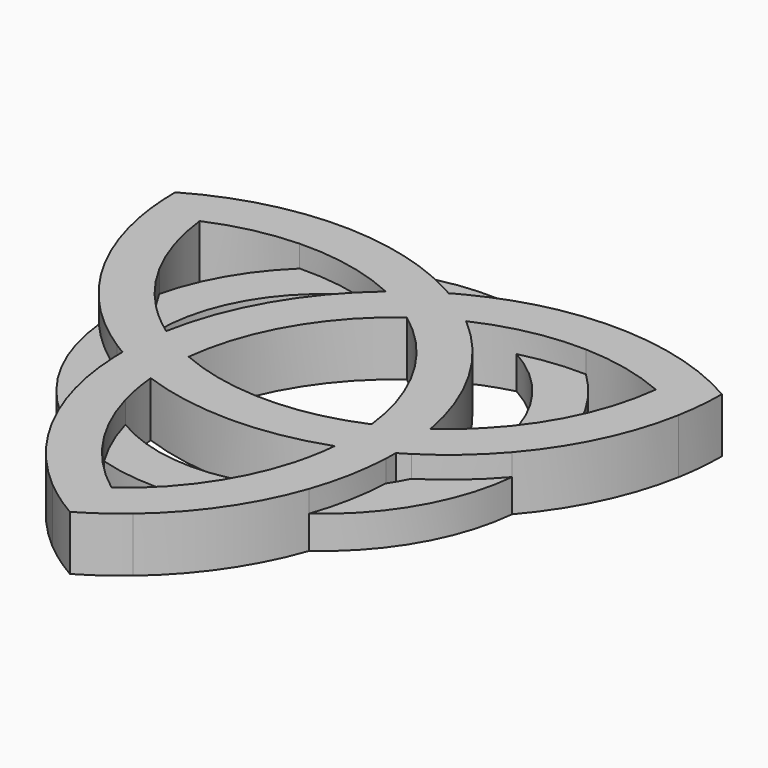
from build123d import *

# Parameters (mm, degrees)
F1_DEPTH = 5
F2_DEPTH = 3


with BuildPart() as f1:
    # F0 (on Top) → F1 (new body)
    with BuildSketch(Plane.XY):
        with BuildLine():
            ThreePointArc((24.5947175074, 9.9504687923), (24.8984732231, 12.1829721649), (25, 14.4337567297))
            ThreePointArc((25, 14.4337567297), (23, 15.4712242442), (20.9147175074, 16.3244157642))
            ThreePointArc((20.9147175074, 16.3244157642), (20.9786685428, 15.3800474736), (21, 14.4337567297))
            ThreePointArc((21, 14.4337567297), (20.9659167777, 13.237791149), (20.8637777457, 12.0457076978))
            ThreePointArc((20.8637777457, 12.0457076978), (22.7827532073, 11.0933643008), (24.5947175074, 9.9504687923))
        make_face()
        with BuildLine():
            ThreePointArc((18.901890558, -1.9283498991), (22.544740222, 3.6293739003), (24.5947175074, 9.9504687923))
            ThreePointArc((24.5947175074, 9.9504687923), (22.7827532073, 11.0933643008), (20.8637777457, 12.0457076978))
            ThreePointArc((20.8637777457, 12.0457076978), (20.0319225906, 8.1312114245), (18.4725923104, 4.4455970728))
            ThreePointArc((18.4725923104, 4.4455970728), (18.8676873768, 2.2383862605), (19, 0))
            ThreePointArc((19, 0), (18.9754567877, -0.9654220315), (18.901890558, -1.9283498991))
        make_face()
        with BuildLine():
            ThreePointArc((13.4505266316, -6.6395280957), (16.3468200119, -4.4813556278), (18.901890558, -1.9283498991))
            ThreePointArc((18.901890558, -1.9283498991), (18.9754567877, -0.9654220315), (19, 0))
            ThreePointArc((19, 0), (18.8676873768, 2.2383862605), (18.4725923104, 4.4455970728))
            ThreePointArc((18.4725923104, 4.4455970728), (16.900090485, 1.9683268696), (14.9976487046, -0.2655811238))
            ThreePointArc((14.9976487046, -0.2655811238), (14.5767441491, -3.5381534747), (13.4505266316, -6.6395280957))
        make_face()
        with BuildLine():
            ThreePointArc((12.5, -7.2168783649), (12.9784741571, -6.9334894324), (13.4505266316, -6.6395280957))
            ThreePointArc((13.4505266316, -6.6395280957), (14.5767441491, -3.5381534747), (14.9976487046, -0.2655811238))
            ThreePointArc((14.9976487046, -0.2655811238), (13.6022734946, -1.5655606237), (12.0947175074, -2.7335904275))
            ThreePointArc((12.0947175074, -2.7335904275), (12.3984732231, -4.9660938001), (12.5, -7.2168783649))
        make_face()
        with BuildLine():
            ThreePointArc((8.4147175074, -9.1075373993), (10.5, -8.2543458793), (12.5, -7.2168783649))
            ThreePointArc((12.5, -7.2168783649), (12.3984732231, -4.9660938001), (12.0947175074, -2.7335904275))
            ThreePointArc((12.0947175074, -2.7335904275), (10.2827532073, -3.876485936), (8.3637777457, -4.8288293329))
            ThreePointArc((8.3637777457, -4.8288293329), (8.4659167777, -6.0209127841), (8.5, -7.2168783649))
            ThreePointArc((8.5, -7.2168783649), (8.4786685428, -8.1631691088), (8.4147175074, -9.1075373993))
        make_face()
        with BuildLine():
            ThreePointArc((-8.4147175074, -9.1075373993), (0, -10.5662432703), (8.4147175074, -9.1075373993))
            ThreePointArc((8.4147175074, -9.1075373993), (8.4786685428, -8.1631691088), (8.5, -7.2168783649))
            ThreePointArc((8.5, -7.2168783649), (8.4659167777, -6.0209127841), (8.3637777457, -4.8288293329))
            ThreePointArc((8.3637777457, -4.8288293329), (0, -6.5662432703), (-8.3637777457, -4.8288293329))
            ThreePointArc((-8.3637777457, -4.8288293329), (-8.4985119016, -6.9668825304), (-8.4147175074, -9.1075373993))
        make_face()
        with BuildLine():
            ThreePointArc((-12.0947175074, -2.7335904275), (-12.3984732231, -4.9660938001), (-12.5, -7.2168783649))
            ThreePointArc((-12.5, -7.2168783649), (-10.5, -8.2543458793), (-8.4147175074, -9.1075373993))
            ThreePointArc((-8.4147175074, -9.1075373993), (-8.4985119016, -6.9668825304), (-8.3637777457, -4.8288293329))
            ThreePointArc((-8.3637777457, -4.8288293329), (-10.2827532073, -3.876485936), (-12.0947175074, -2.7335904275))
        make_face()
        with BuildLine():
            ThreePointArc((-14.9976487046, -0.2655811238), (-14.5767441491, -3.5381534747), (-13.4505266316, -6.6395280957))
            ThreePointArc((-13.4505266316, -6.6395280957), (-12.9784741571, -6.9334894324), (-12.5, -7.2168783649))
            ThreePointArc((-12.5, -7.2168783649), (-12.3984732231, -4.9660938001), (-12.0947175074, -2.7335904275))
            ThreePointArc((-12.0947175074, -2.7335904275), (-13.6022734946, -1.5655606237), (-14.9976487046, -0.2655811238))
        make_face()
        with BuildLine():
            ThreePointArc((-18.4725923104, 4.4455970728), (-18.9570512586, 1.2767958254), (-18.901890558, -1.9283498991))
            ThreePointArc((-18.901890558, -1.9283498991), (-16.3468200119, -4.4813556278), (-13.4505266316, -6.6395280957))
            ThreePointArc((-13.4505266316, -6.6395280957), (-14.5767441491, -3.5381534747), (-14.9976487046, -0.2655811238))
            ThreePointArc((-14.9976487046, -0.2655811238), (-16.900090485, 1.9683268696), (-18.4725923104, 4.4455970728))
        make_face()
        with BuildLine():
            ThreePointArc((-20.8637777457, 12.0457076978), (-22.7827532073, 11.0933643008), (-24.5947175074, 9.9504687923))
            ThreePointArc((-24.5947175074, 9.9504687923), (-22.544740222, 3.6293739003), (-18.901890558, -1.9283498991))
            ThreePointArc((-18.901890558, -1.9283498991), (-18.9570512586, 1.2767958254), (-18.4725923104, 4.4455970728))
            ThreePointArc((-18.4725923104, 4.4455970728), (-20.0319225906, 8.1312114245), (-20.8637777457, 12.0457076978))
        make_face()
        with BuildLine():
            ThreePointArc((-20.9147175074, 16.3244157642), (-23, 15.4712242442), (-25, 14.4337567297))
            ThreePointArc((-25, 14.4337567297), (-24.8984732231, 12.1829721649), (-24.5947175074, 9.9504687923))
            ThreePointArc((-24.5947175074, 9.9504687923), (-22.7827532073, 11.0933643008), (-20.8637777457, 12.0457076978))
            ThreePointArc((-20.8637777457, 12.0457076978), (-20.9985119016, 14.1837608953), (-20.9147175074, 16.3244157642))
        make_face()
        with BuildLine():
            ThreePointArc((-7.780945279, 17.3336923523), (-14.4155001085, 17.7096308038), (-20.9147175074, 16.3244157642))
            ThreePointArc((-20.9147175074, 16.3244157642), (-20.9985119016, 14.1837608953), (-20.8637777457, 12.0457076978))
            ThreePointArc((-20.8637777457, 12.0457076978), (-17.0577969525, 13.2825481378), (-13.0862961552, 13.7749356782))
            ThreePointArc((-13.0862961552, 13.7749356782), (-10.5842632495, 15.7788900581), (-7.780945279, 17.3336923523))
        make_face()
        with BuildLine():
            ThreePointArc((-0.9752633158, 14.9682618051), (-4.2924421889, 16.3974392153), (-7.780945279, 17.3336923523))
            ThreePointArc((-7.780945279, 17.3336923523), (-10.5842632495, 15.7788900581), (-13.0862961552, 13.7749356782))
            ThreePointArc((-13.0862961552, 13.7749356782), (-10.1546663145, 13.6517442515), (-7.2688243523, 13.1211353371))
            ThreePointArc((-7.2688243523, 13.1211353371), (-4.224241283, 14.392907475), (-0.9752633158, 14.9682618051))
        make_face()
        with BuildLine():
            ThreePointArc((0, 14.4337567297), (-0.4846590933, 14.7064330386), (-0.9752633158, 14.9682618051))
            ThreePointArc((-0.9752633158, 14.9682618051), (-4.224241283, 14.392907475), (-7.2688243523, 13.1211353371))
            ThreePointArc((-7.2688243523, 13.1211353371), (-5.445321476, 12.5626947074), (-3.68, 11.8411278268))
            ThreePointArc((-3.68, 11.8411278268), (-1.8984732231, 13.2204396794), (0, 14.4337567297))
        make_face()
        with BuildLine():
            ThreePointArc((3.68, 11.8411278268), (1.8984732231, 13.2204396794), (0, 14.4337567297))
            ThreePointArc((0, 14.4337567297), (-1.8984732231, 13.2204396794), (-3.68, 11.8411278268))
            ThreePointArc((-3.68, 11.8411278268), (-1.7842413057, 10.8433684664), (0, 9.6576586658))
            ThreePointArc((0, 9.6576586658), (1.7842413057, 10.8433684664), (3.68, 11.8411278268))
        make_face()
        with BuildLine():
            ThreePointArc((8.3637777457, -4.8288293329), (10.2827532073, -3.876485936), (12.0947175074, -2.7335904275))
            ThreePointArc((12.0947175074, -2.7335904275), (9.1506350946, 5.2831216351), (3.68, 11.8411278268))
            ThreePointArc((3.68, 11.8411278268), (1.7842413057, 10.8433684664), (0, 9.6576586658))
            ThreePointArc((0, 9.6576586658), (5.6865334795, 3.2831216351), (8.3637777457, -4.8288293329))
        make_face()
        with BuildLine():
            ThreePointArc((12.4752633158, -8.3287337094), (12.4938150639, -7.7729436062), (12.5, -7.2168783649))
            ThreePointArc((12.5, -7.2168783649), (10.5, -8.2543458793), (8.4147175074, -9.1075373993))
            ThreePointArc((8.4147175074, -9.1075373993), (8.1569520186, -10.9971340837), (7.7288243523, -12.8555542133))
            ThreePointArc((7.7288243523, -12.8555542133), (10.3525028661, -10.8547540003), (12.4752633158, -8.3287337094))
        make_face()
        with BuildLine():
            ThreePointArc((5.3862961552, -18.2205327509), (8.3727880091, -17.0556858835), (11.120945279, -15.4053424532))
            ThreePointArc((11.120945279, -15.4053424532), (12.054377823, -11.9160835875), (12.4752633158, -8.3287337094))
            ThreePointArc((12.4752633158, -8.3287337094), (10.3525028661, -10.8547540003), (7.7288243523, -12.8555542133))
            ThreePointArc((7.7288243523, -12.8555542133), (6.7454241705, -15.620071121), (5.3862961552, -18.2205327509))
        make_face()
        with BuildLine():
            ThreePointArc((0, -24.0914153956), (1.7842413057, -25.2771251961), (3.68, -26.2748845565))
            ThreePointArc((3.68, -26.2748845565), (8.1292401135, -21.3390047041), (11.120945279, -15.4053424532))
            ThreePointArc((11.120945279, -15.4053424532), (8.3727880091, -17.0556858835), (5.3862961552, -18.2205327509))
            ThreePointArc((5.3862961552, -18.2205327509), (2.9741256381, -21.4137595623), (0, -24.0914153956))
        make_face()
        with BuildLine():
            ThreePointArc((-3.68, -26.2748845565), (-1.8984732231, -27.6541964091), (0, -28.8675134595))
            ThreePointArc((0, -28.8675134595), (1.8984732231, -27.6541964091), (3.68, -26.2748845565))
            ThreePointArc((3.68, -26.2748845565), (1.7842413057, -25.2771251961), (0, -24.0914153956))
            ThreePointArc((0, -24.0914153956), (-1.7842413057, -25.2771251961), (-3.68, -26.2748845565))
        make_face()
        with BuildLine():
            ThreePointArc((-11.120945279, -15.4053424532), (-8.1292401135, -21.3390047041), (-3.68, -26.2748845565))
            ThreePointArc((-3.68, -26.2748845565), (-1.7842413057, -25.2771251961), (0, -24.0914153956))
            ThreePointArc((0, -24.0914153956), (-2.9741256381, -21.4137595624), (-5.3862961552, -18.220532751))
            ThreePointArc((-5.3862961552, -18.2205327509), (-8.3727880091, -17.0556858835), (-11.120945279, -15.4053424532))
        make_face()
        with BuildLine():
            ThreePointArc((-12.4752633158, -8.3287337094), (-12.054377823, -11.9160835875), (-11.120945279, -15.4053424532))
            ThreePointArc((-11.120945279, -15.4053424532), (-8.3727880091, -17.0556858835), (-5.3862961552, -18.2205327509))
            ThreePointArc((-5.3862961552, -18.220532751), (-6.7454241705, -15.620071121), (-7.7288243523, -12.8555542133))
            ThreePointArc((-7.7288243523, -12.8555542133), (-10.3525028661, -10.8547540003), (-12.4752633158, -8.3287337094))
        make_face()
        with BuildLine():
            ThreePointArc((-8.4147175074, -9.1075373993), (-10.5, -8.2543458793), (-12.5, -7.2168783649))
            ThreePointArc((-12.5, -7.2168783649), (-12.4938150639, -7.7729436062), (-12.4752633158, -8.3287337094))
            ThreePointArc((-12.4752633158, -8.3287337094), (-10.3525028661, -10.8547540003), (-7.7288243523, -12.8555542133))
            ThreePointArc((-7.7288243523, -12.8555542133), (-8.1569520186, -10.9971340837), (-8.4147175074, -9.1075373993))
        make_face()
        with BuildLine():
            ThreePointArc((0, 9.6576586658), (-1.7842413057, 10.8433684664), (-3.68, 11.8411278268))
            ThreePointArc((-3.68, 11.8411278268), (-9.1506350946, 5.2831216351), (-12.0947175074, -2.7335904275))
            ThreePointArc((-12.0947175074, -2.7335904275), (-10.2827532073, -3.876485936), (-8.3637777457, -4.8288293329))
            ThreePointArc((-8.3637777457, -4.8288293329), (-5.6865334795, 3.2831216351), (0, 9.6576586658))
        make_face()
        with BuildLine():
            ThreePointArc((7.2688243523, 13.1211353371), (4.224241283, 14.392907475), (0.9752633158, 14.9682618051))
            ThreePointArc((0.9752633158, 14.9682618051), (0.4846590933, 14.7064330386), (0, 14.4337567297))
            ThreePointArc((0, 14.4337567297), (1.8984732231, 13.2204396794), (3.68, 11.8411278268))
            ThreePointArc((3.68, 11.8411278268), (5.445321476, 12.5626947074), (7.2688243523, 13.1211353371))
        make_face()
        with BuildLine():
            ThreePointArc((13.0862961552, 13.7749356782), (10.5842632495, 15.7788900581), (7.780945279, 17.3336923523))
            ThreePointArc((7.780945279, 17.3336923523), (4.2924421889, 16.3974392153), (0.9752633158, 14.9682618051))
            ThreePointArc((0.9752633158, 14.9682618051), (4.224241283, 14.392907475), (7.2688243523, 13.1211353371))
            ThreePointArc((7.2688243523, 13.1211353371), (10.1546663145, 13.6517442515), (13.0862961552, 13.7749356782))
        make_face()
        with BuildLine():
            ThreePointArc((21, 14.4337567297), (20.9786685428, 15.3800474736), (20.9147175074, 16.3244157642))
            ThreePointArc((20.9147175074, 16.3244157642), (14.4155001085, 17.7096308038), (7.780945279, 17.3336923523))
            ThreePointArc((7.780945279, 17.3336923523), (10.5842632495, 15.7788900581), (13.0862961552, 13.7749356782))
            ThreePointArc((13.0862961552, 13.7749356782), (17.0577969525, 13.2825481378), (20.8637777457, 12.0457076978))
            ThreePointArc((20.8637777457, 12.0457076978), (20.9659167777, 13.237791149), (21, 14.4337567297))
        make_face()
    extrude(amount=F1_DEPTH)

    # F0 (on Top) → F2 (join)
    with BuildSketch(Plane.XY):
        with BuildLine():
            ThreePointArc((0.9752633158, 14.9682618051), (4.2924421889, 16.3974392153), (7.780945279, 17.3336923523))
            ThreePointArc((7.780945279, 17.3336923523), (0, 19), (-7.780945279, 17.3336923523))
            ThreePointArc((-7.780945279, 17.3336923523), (-4.2924421889, 16.3974392153), (-0.9752633158, 14.9682618051))
            ThreePointArc((-0.9752633158, 14.9682618051), (0, 15), (0.9752633158, 14.9682618051))
        make_face()
        with BuildLine():
            ThreePointArc((14.9976487046, -0.2655811238), (16.900090485, 1.9683268696), (18.4725923104, 4.4455970728))
            ThreePointArc((18.4725923104, 4.4455970728), (16.4544826719, 9.5), (13.0862961552, 13.7749356782))
            ThreePointArc((13.0862961552, 13.7749356782), (10.1546663145, 13.6517442515), (7.2688243523, 13.1211353371))
            ThreePointArc((7.2688243523, 13.1211353371), (12.9234740934, 7.6147105892), (15, 0))
            ThreePointArc((15, 0), (14.9994121646, -0.132795766), (14.9976487046, -0.2655811238))
        make_face()
        with BuildLine():
            ThreePointArc((11.120945279, -15.4053424532), (16.4544826719, -9.5), (18.901890558, -1.9283498991))
            ThreePointArc((18.901890558, -1.9283498991), (16.3468200119, -4.4813556278), (13.4505266316, -6.6395280957))
            ThreePointArc((13.4505266316, -6.6395280957), (12.9903810568, -7.5), (12.4752633158, -8.3287337094))
            ThreePointArc((12.4752633158, -8.3287337094), (12.054377823, -11.9160835875), (11.120945279, -15.4053424532))
        make_face()
        with BuildLine():
            ThreePointArc((-5.3862961552, -18.2205327509), (0, -19), (5.3862961552, -18.2205327509))
            ThreePointArc((5.3862961552, -18.2205327509), (6.7454241705, -15.620071121), (7.7288243523, -12.8555542133))
            ThreePointArc((7.7288243523, -12.8555542133), (0, -15), (-7.7288243523, -12.8555542133))
            ThreePointArc((-7.7288243523, -12.8555542133), (-6.7454241705, -15.620071121), (-5.3862961552, -18.220532751))
        make_face()
        with BuildLine():
            ThreePointArc((-13.4505266316, -6.6395280957), (-16.3468200119, -4.4813556278), (-18.901890558, -1.9283498991))
            ThreePointArc((-18.901890558, -1.9283498991), (-16.4544826719, -9.5), (-11.120945279, -15.4053424532))
            ThreePointArc((-11.120945279, -15.4053424532), (-12.054377823, -11.9160835875), (-12.4752633158, -8.3287337094))
            ThreePointArc((-12.4752633158, -8.3287337094), (-12.9903810568, -7.5), (-13.4505266316, -6.6395280957))
        make_face()
        with BuildLine():
            ThreePointArc((-13.0862961552, 13.7749356782), (-16.4544826719, 9.5), (-18.4725923104, 4.4455970728))
            ThreePointArc((-18.4725923104, 4.4455970728), (-16.900090485, 1.9683268696), (-14.9976487046, -0.2655811238))
            ThreePointArc((-14.9976487046, -0.2655811238), (-12.9903810568, 7.5), (-7.2688243523, 13.1211353371))
            ThreePointArc((-7.2688243523, 13.1211353371), (-10.1546663145, 13.6517442515), (-13.0862961552, 13.7749356782))
        make_face()
    extrude(amount=F2_DEPTH)


solid = f1.part
